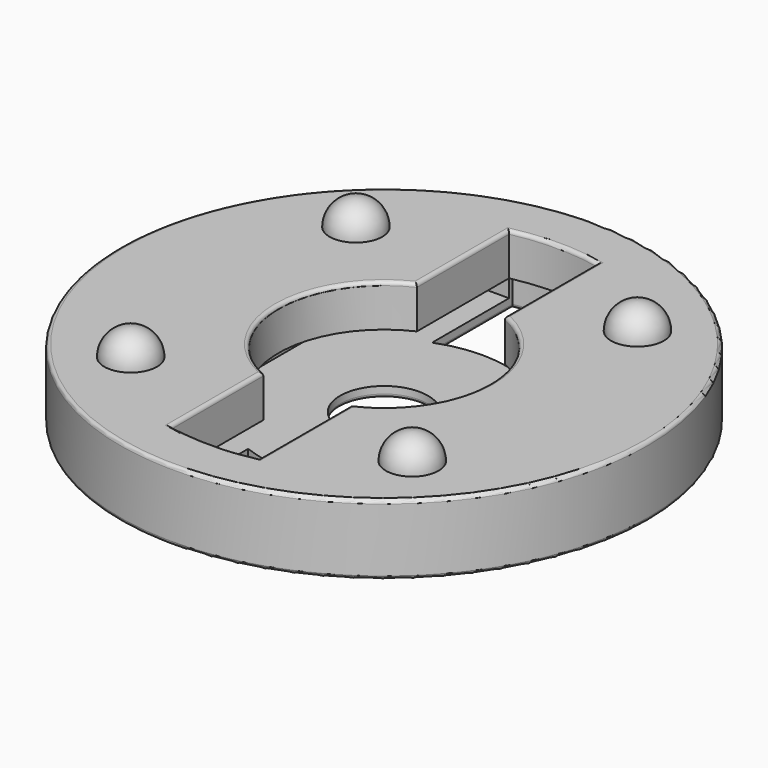
from build123d import *

# Parameters (mm, degrees)
F0_R          = 95.25
F1_DEPTH      = 12.7
F1_DEPTH_BACK = 12.7
F3_DEPTH      = 15.24
F4_R          = 1.27
F5_W          = 88.9
F5_H          = 6.35
F6_DEPTH      = 76.2
F6_DEPTH_BACK = 76.2
F7_R          = 9.525
F8_DEPTH      = 9.525
F9_R          = 9.52499
F10_R         = 15.875
F11_DEPTH     = 10.16
F12_R         = 1.27


# Not quite as in the source:
# - a fillet or chamfer is up to 0.001 mm smaller than in the source, because OpenCascade refuses the exact size


with BuildPart() as f1:
    # F0 (on Top) → F1 (new body, two sides)
    with BuildSketch(Plane.XY) as f1_sk:
        Circle(F0_R)
    extrude(amount=-F1_DEPTH)
    extrude(f1_sk.sketch, amount=F1_DEPTH_BACK)

    # F2 (on face) → F3 (cut)
    with BuildSketch(Plane.XY.offset(12.7)):
        with BuildLine():
            Line((-15.875, -34.635160964), (-15.875, 34.635160964))
            ThreePointArc((-15.875, 34.635160964), (-38.1, 0), (-15.875, -34.635160964))
        make_face()
        Polygon((-15.875, 76.2), (-15.875, 34.635160964), (-15.875, -34.635160964), (-15.875, -76.2), (15.875, -76.2), (15.875, -34.635160964), (15.875, 34.635160964), (15.875, 76.2), align=None)
        with BuildLine():
            ThreePointArc((15.875, 76.2), (0, 77.8439802245), (-15.875, 76.2))
            Line((-15.875, 76.2), (15.875, 76.2))
        make_face()
        with BuildLine():
            Line((15.875, -76.2), (-15.875, -76.2))
            ThreePointArc((-15.875, -76.2), (0, -77.8439802245), (15.875, -76.2))
        make_face()
        with BuildLine():
            ThreePointArc((15.875, -34.635160964), (38.1, 0), (15.875, 34.635160964))
            Line((15.875, 34.635160964), (15.875, -34.635160964))
        make_face()
    extrude(amount=-F3_DEPTH, mode=Mode.SUBTRACT)

    # F4
    f4_edges = [f1.edges().sort_by_distance(p)[0] for p in [
        (-95.25, 0, 12.7),
        (-38.1, 0, 12.7),
        (-15.875, -55.41758, 12.7),
        (0, -77.84398, 12.7),
        (15.875, -55.41758, 12.7),
        (38.1, 0, 12.7),
        (15.875, 55.41758, 12.7),
        (0, 77.84398, 12.7),
        (-15.875, 55.41758, 12.7),
        (-95.25, 0, -12.7),
    ]]
    fillet(f4_edges, radius=F4_R)

    # F5 (on Front) → F6 (cut, two sides)
    with BuildSketch(Plane.XZ) as f6_sk:
        with Locations((0, -5.715)):
            Rectangle(F5_W, F5_H)
    extrude(amount=-F6_DEPTH, mode=Mode.SUBTRACT)
    extrude(f6_sk.sketch, amount=F6_DEPTH_BACK, mode=Mode.SUBTRACT)

    # F7 (on face) → F8 (join)
    with BuildSketch(Plane.XY.offset(12.7)):
        with Locations((-50.8, 50.8)):
            Circle(F7_R)
        with Locations((50.8, 50.8)):
            Circle(F7_R)
        with Locations((50.8, -50.8)):
            Circle(F7_R)
        with Locations((-50.8, -50.8)):
            Circle(F7_R)
    extrude(amount=F8_DEPTH)

    # F9 (radius 9.525 in the source; OpenCascade refuses exactly that, so slightly less here)
    f9_edges = [f1.edges().sort_by_distance(p)[0] for p in [
        (-60.325, 50.8, 22.225),
        (41.275, 50.8, 22.225),
        (41.275, -50.8, 22.225),
        (-60.325, -50.8, 22.225),
    ]]
    fillet(f9_edges, radius=F9_R)

    # F10 (on face) → F11 (cut)
    with BuildSketch(Plane(origin=(0, 0, -12.7), x_dir=(1, 0, 0), z_dir=(0, 0, -1))):
        with BuildLine():
            ThreePointArc((-15.875, -77.7712993334), (0, -79.375), (15.875, -77.7712993334))
            Line((15.875, -77.7712993334), (15.875, -41.5185124372))
            ThreePointArc((15.875, -41.5185124372), (0, -44.45), (-15.875, -41.5185124372))
            Line((-15.875, -41.5185124372), (-15.875, -77.7712993334))
        make_face()
        Circle(F10_R)
        with BuildLine():
            Line((-15.875, 77.7712993334), (-15.875, 41.5185124372))
            ThreePointArc((-15.875, 41.5185124372), (0, 44.45), (15.875, 41.5185124372))
            Line((15.875, 41.5185124372), (15.875, 77.7712993334))
            ThreePointArc((15.875, 77.7712993334), (0, 79.375), (-15.875, 77.7712993334))
        make_face()
    extrude(amount=-F11_DEPTH, mode=Mode.SUBTRACT)

    # F12
    f12_edges = [f1.edges().sort_by_distance(p)[0] for p in [
        (-93.98, 0, -12.7),
        (0, -79.375, -12.7),
        (15.875, -59.644906, -12.7),
        (0, -44.45, -12.7),
        (-15.875, -59.644906, -12.7),
        (-15.875, 0, -12.7),
        (15.875, 59.644906, -12.7),
        (0, 79.375, -12.7),
        (-15.875, 59.644906, -12.7),
        (0, 44.45, -12.7),
    ]]
    fillet(f12_edges, radius=F12_R)


solid = f1.part
